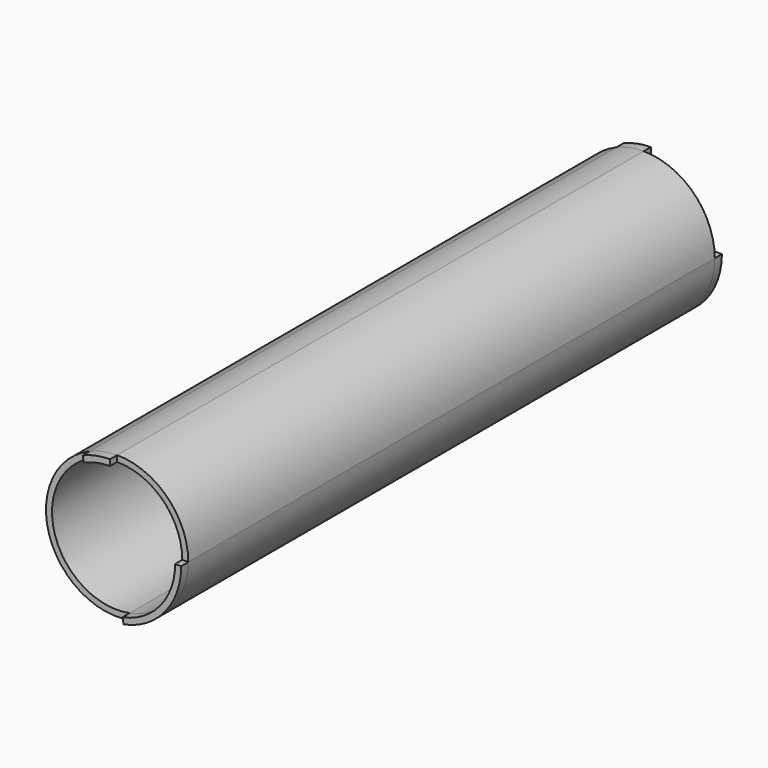
from build123d import *
from build123d import SkipClean  # not in build123d's __all__

# Parameters (mm, degrees)
F1_DEPTH      = 469.9
F3_DEPTH      = 6.35
F3_DEPTH_BACK = 476.25


with BuildPart() as f1:
    # F0 (on Front) → F1 (new body)
    with BuildSketch(Plane.XZ):
        with BuildLine():
            ThreePointArc((0, 46.4007208579), (32.8677374031, 32.786458261), (46.482, -0.0812791421))
            ThreePointArc((46.482, -0.0812791421), (-25.4350635734, -38.9867268971), (-18.6457425678, 42.4970323333))
            Line((-18.6457425678, 42.4970323333), (-19.5480847725, 46.8070177104))
            ThreePointArc((-19.5480847725, 46.8070177104), (-28.1744325014, -42.3523254175), (50.8, -0.0812791421))
            ThreePointArc((50.8, -0.0812791421), (35.9210244843, 35.8397453422), (0, 50.7187208579))
            Line((0, 50.7187208579), (0, 46.4007208579))
        make_face()
        with BuildLine():
            ThreePointArc((-18.6457425678, 42.4970323333), (-9.525, 45.4143327232), (0, 46.4007208579))
            Line((0, 46.4007208579), (0, 50.7187208579))
            ThreePointArc((0, 50.7187208579), (-9.9678111914, 49.731196605), (-19.5480847725, 46.8070177104))
            Line((-19.5480847725, 46.8070177104), (-18.6457425678, 42.4970323333))
        make_face()
    extrude(amount=F1_DEPTH)

    # F2 (on face) → F3 (join, two sides)
    with BuildSketch(Plane(origin=(0, 0, 0), x_dir=(-1, 0, 0), z_dir=(0, 1, 0))) as f3_sk:
        with BuildLine():
            ThreePointArc((19.5480847725, 46.8070177104), (9.9678111914, 49.731196605), (0, 50.7187208579))
            Line((0, 50.7187208579), (0, 46.4007208579))
            ThreePointArc((0, 46.4007208579), (9.525, 45.4143327232), (18.6457425678, 42.4970323333))
            Line((18.6457425678, 42.4970323333), (19.5480847725, 46.8070177104))
        make_face()
        with BuildLine():
            Line((-46.481928937, 0), (-50.7999349773, 0))
            ThreePointArc((-50.7999349773, 0), (-39.2292934041, -32.3566960877), (-9.7083203647, -49.9449785205))
            Line((-9.7083203647, -49.9449785205), (-8.8844070807, -45.7063121265))
            ThreePointArc((-8.8844070807, -45.7063121265), (-35.897416802, -29.610108969), (-46.481928937, 0))
        make_face()
    with SkipClean():  # cleaning this boolean's faces spoils the solid; the shape is the same uncleaned
        extrude(amount=F3_DEPTH)
        extrude(f3_sk.sketch, amount=-F3_DEPTH_BACK)


solid = f1.part
